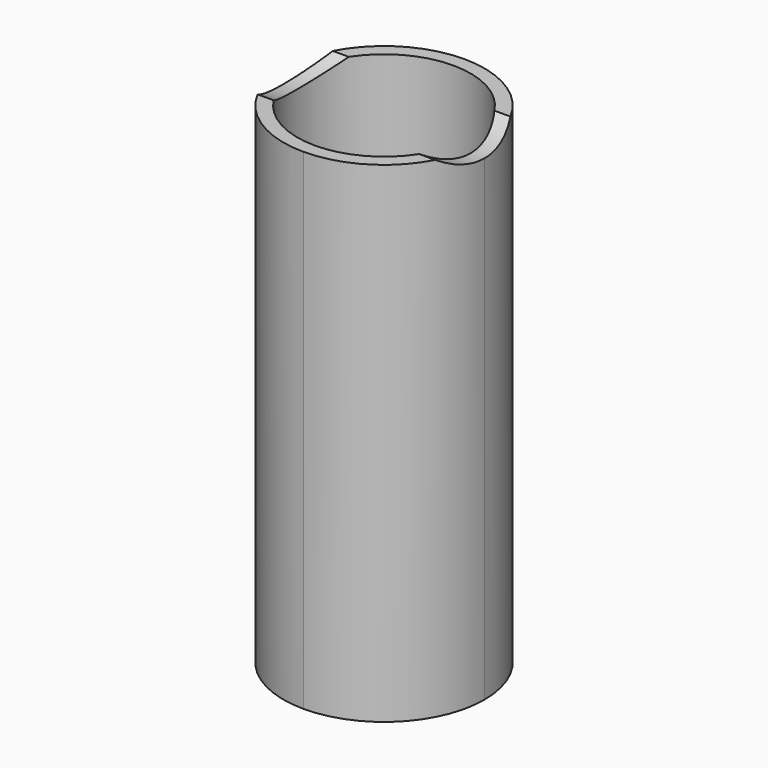
from build123d import *

# Parameters (mm, degrees)
F0_W     = 3.683
F0_H     = 3.683
F0_R     = 1.5875
F1_DEPTH = 8.98525
F3_DEPTH = 3.683
F4_R     = 1.84149


# Not quite as in the source:
# - a fillet or chamfer is up to 0.001 mm smaller than in the source, because OpenCascade refuses the exact size


with BuildPart() as f1:
    # F0 (on Top) → F1 (new body)
    with BuildSketch(Plane.XY):
        Rectangle(F0_W, F0_H)
        Circle(F0_R, mode=Mode.SUBTRACT)
    extrude(amount=F1_DEPTH)

    # F2 (on face) → F3 (cut, through all)
    with BuildSketch(Plane.YZ.offset(1.8415)):
        with BuildLine():
            Line((0.8613559079, 8.98525), (-0.8613559079, 8.98525))
            ThreePointArc((-0.8613559079, 8.98525), (0, 8.73125), (0.8613559079, 8.98525))
        make_face()
    extrude(amount=-F3_DEPTH, mode=Mode.SUBTRACT)

    # F4 (radius 1.8415 in the source; OpenCascade refuses exactly that, so slightly less here)
    f4_edges = [f1.edges().sort_by_distance(p)[0] for p in [
        (-1.8415, -1.8415, 4.492625),
        (1.8415, -1.8415, 4.492625),
        (-1.8415, 1.8415, 4.492625),
        (1.8415, 1.8415, 4.492625),
    ]]
    fillet(f4_edges, radius=F4_R)


solid = f1.part
